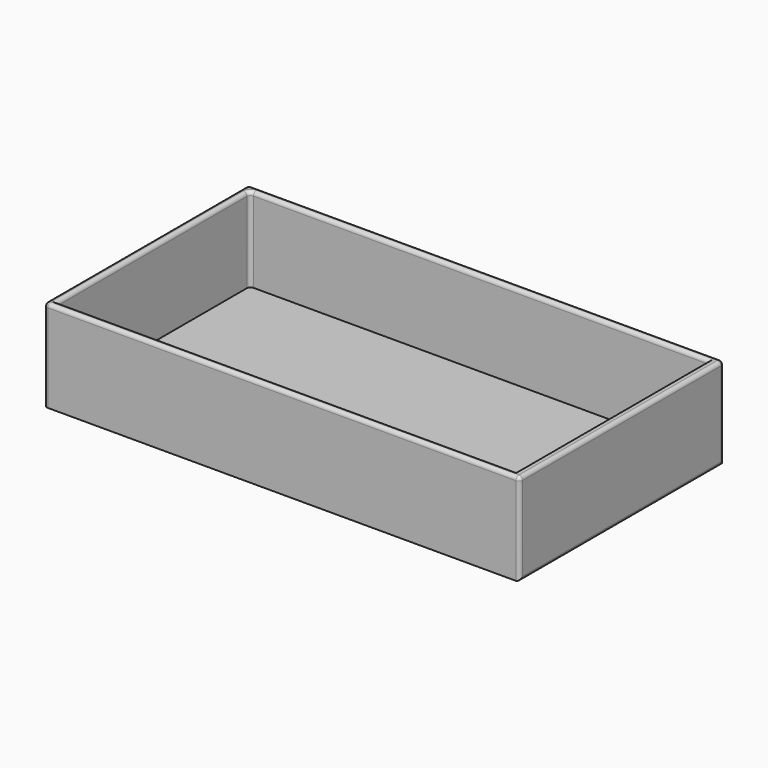
from build123d import *

# Parameters (mm, degrees)
F0_W     = 129.5
F0_H     = 69.5
F1_DEPTH = 25
F2_T     = -2
F3_R     = 0.99999


# Not quite as in the source:
# - a fillet or chamfer is up to 0.001 mm smaller than in the source, because OpenCascade refuses the exact size


with BuildPart() as f1:
    # F0 (on Top) → F1 (new body)
    with BuildSketch(Plane.XY):
        with Locations((8.1922735609, -6.6703366488)):
            Rectangle(F0_W, F0_H)
    extrude(amount=F1_DEPTH)

    # F2
    f2_openings = [f1.faces().sort_by_distance(p)[0] for p in [
        (8.192274, -6.670337, 25),
    ]]
    offset(amount=F2_T, openings=f2_openings)

    # F3 (radius 1 in the source; OpenCascade refuses exactly that, so slightly less here)
    f3_edges = [f1.edges().sort_by_distance(p)[0] for p in [
        (8.192274, 26.079663, 25),
        (-56.557726, -6.670337, 25),
        (-54.557726, -6.670337, 25),
        (8.192274, -41.420337, 25),
        (72.942274, -6.670337, 0),
        (72.942274, -6.670337, 25),
        (8.192274, -39.420337, 25),
        (8.192274, 28.079663, 25),
        (72.942274, 28.079663, 12.5),
        (-56.557726, 28.079663, 12.5),
        (-56.557726, -41.420337, 12.5),
        (-54.557726, 26.079663, 13.5),
        (72.942274, -41.420337, 12.5),
    ]]
    fillet(f3_edges, radius=F3_R)


solid = f1.part
